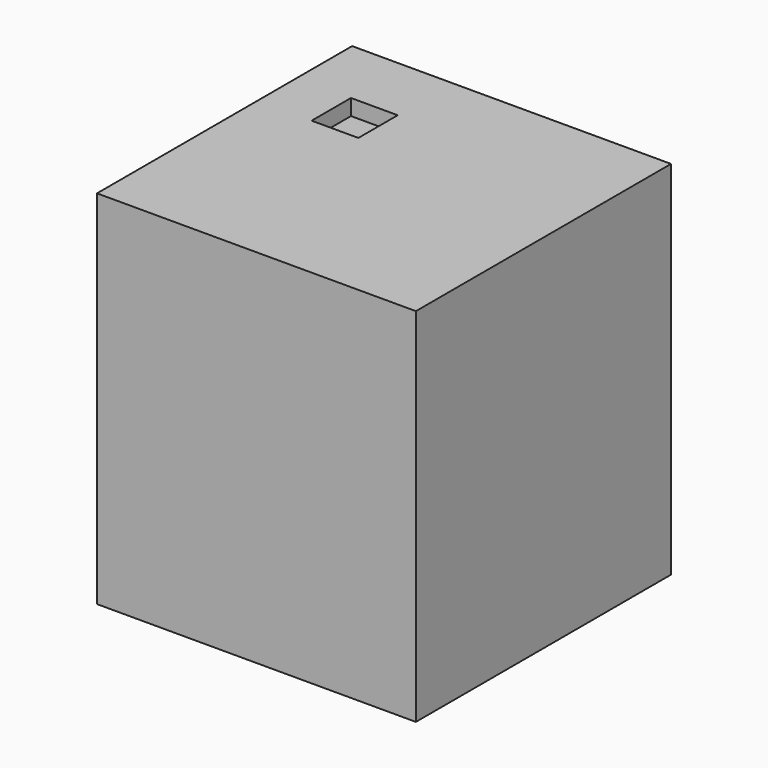
from build123d import *

# Parameters (mm, degrees)
F1_W      = 2540
F1_H      = 2540
F2_DEPTH  = 1270
F3_W      = 372.1394836903
F3_H      = 391.725808382
F4_DEPTH  = 127
F5_W      = 2540
F5_H      = 2540
F5_W_2    = 372.1394836903
F5_H_2    = 391.725808382
F6_DEPTH  = 127
F7_DEPTH  = 127
F8_DEPTH  = 127
F6_FACE_W = 2540
F6_FACE_H = 2540
F9_DEPTH  = 213.36


# Not quite as in the source:
# - a variable given as a bare number and used for a length is read in inches; the dataset says mm whatever the document's units were


with BuildPart() as f2:
    # F1 (on Front) → F2 (new body, symmetric)
    with BuildSketch(Plane.XZ):
        Rectangle(F1_W, F1_H)
    extrude(amount=F2_DEPTH, both=True)

    # F3 (on face) → F4 (cut)
    with BuildSketch(Plane.XY.offset(1270)):
        with Locations((-652.8763622046, 523.9332765341)):
            Rectangle(F3_W, F3_H)
    extrude(amount=-F4_DEPTH, mode=Mode.SUBTRACT)

    # F5 (on face) → F6 (join)
    with BuildSketch(Plane(origin=(0, 0, -1270), x_dir=(1, 0, 0), z_dir=(0, 0, -1))):
        Rectangle(F5_W, F5_H)
        with Locations((-652.8763622046, -523.9332765341)):
            Rectangle(F5_W_2, F5_H_2, mode=Mode.SUBTRACT)
        with Locations((-652.8763622046, -523.9332765341)):
            Rectangle(F5_W_2, F5_H_2)
    extrude(amount=F6_DEPTH)

    # F5 (on face) → F7 (join)
    with BuildSketch(Plane(origin=(0, 0, -1270), x_dir=(1, 0, 0), z_dir=(0, 0, -1))):
        with Locations((-652.8763622046, -523.9332765341)):
            Rectangle(F5_W_2, F5_H_2)
    extrude(amount=F7_DEPTH)

    # F5 (on face) → F8 (join)
    with BuildSketch(Plane(origin=(0, 0, -1270), x_dir=(1, 0, 0), z_dir=(0, 0, -1))):
        with Locations((-652.8763622046, -523.9332765341)):
            Rectangle(F5_W_2, F5_H_2)
    extrude(amount=F8_DEPTH)

    # F5 (on face) + F6_face (on face) → F9 (join)
    with BuildSketch(Plane(origin=(0, 0, -1270), x_dir=(1, 0, 0), z_dir=(0, 0, -1))):
        with Locations((-652.8763622046, -523.9332765341)):
            Rectangle(F5_W_2, F5_H_2)
    with BuildSketch(Plane(origin=(0, 0, -1397), x_dir=(1, 0, 0), z_dir=(0, 0, -1))):
        Rectangle(F6_FACE_W, F6_FACE_H)
    extrude(amount=F9_DEPTH)


solid = f2.part
